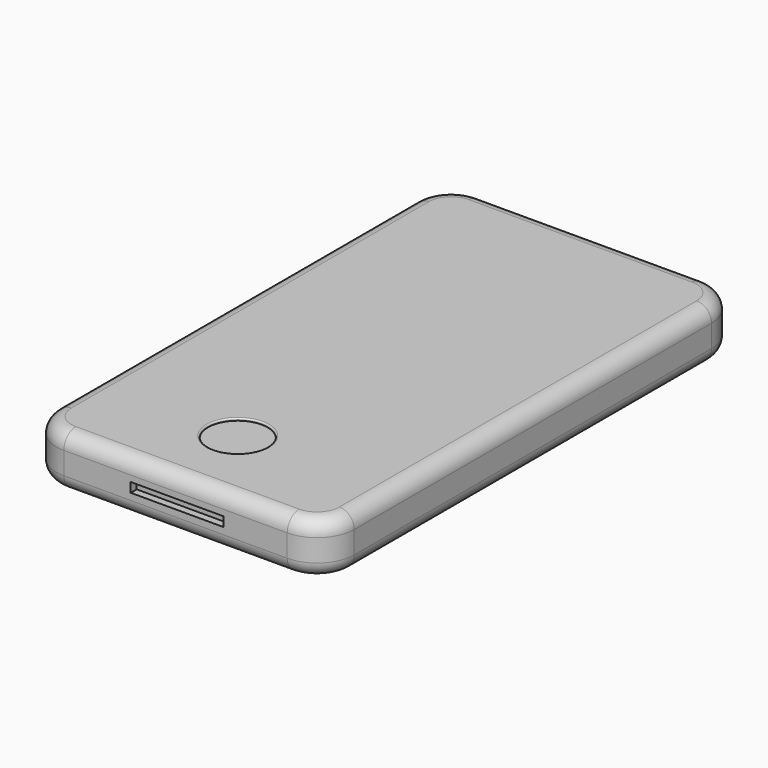
from build123d import *

# Parameters (mm, degrees)
F0_W         = 40
F0_H         = 70
F1_DEPTH     = 7
F2_R         = 5
F3_R         = 2
F4_DEPTH     = 5
F5_T1_DEPTH  = 60
F5_T3_DEPTH  = 30
F5_T6_ANGLE  = 90
F5_T8_ANGLE  = 90
F5_T10_ANGLE = 90
F5_T12_ANGLE = 90
F5_T14_ANGLE = 90
F5_T16_ANGLE = 90
F5_T18_ANGLE = 90
F5_T20_ANGLE = 90
F6_R         = 4
F7_DEPTH     = 0.3
F8_R         = 0.2
F9_W         = 12.4906748533
F9_H         = 1.2735207565
F10_DEPTH    = 1


# Not quite as in the source:
# - a fillet or chamfer that OpenCascade refuses, or shapes differently, is made with other operations: its cross-section is extruded or revolved along the edge and cut away or added


with BuildPart() as f1:
    # F0 (on Top) → F1 (new body)
    with BuildSketch(Plane.XY):
        with Locations((20, 35)):
            Rectangle(F0_W, F0_H)
    extrude(amount=F1_DEPTH)

    # F2
    f2_edges = [f1.edges().sort_by_distance(p)[0] for p in [
        (40, 0, 3.5),
        (0, 0, 3.5),
        (40, 70, 3.5),
        (0, 70, 3.5),
    ]]
    fillet(f2_edges, radius=F2_R)

    # F3 (on face) → F4 (cut)
    with BuildSketch(Plane(origin=(0, 70, 0), x_dir=(-1, 0, 0), z_dir=(0, 1, 0))):
        with Locations((-30.8697689325, 3.5)):
            Circle(F3_R)
    extrude(amount=-F4_DEPTH, mode=Mode.SUBTRACT)

    # F5: fillet of radius 2 on 16 edges, made by hand

    # F5_s2 → F5_t1 (cut)
    with BuildSketch(Plane.XZ.offset(-65)):
        with BuildLine():
            ThreePointArc((0, 5), (0.5857864376, 6.4142135624), (2, 7))
            Line((2, 7), (0, 7))
            Line((0, 7), (0, 5))
        make_face()
        with BuildLine():
            ThreePointArc((38, 7), (39.4142135624, 6.4142135624), (40, 5))
            Line((40, 5), (40, 7))
            Line((40, 7), (38, 7))
        make_face()
        with BuildLine():
            ThreePointArc((0, 2), (0.5857864376, 0.5857864376), (2, 0))
            Line((2, 0), (0, 0))
            Line((0, 0), (0, 2))
        make_face()
        with BuildLine():
            ThreePointArc((38, 0), (39.4142135624, 0.5857864376), (40, 2))
            Line((40, 2), (40, 0))
            Line((40, 0), (38, 0))
        make_face()
    extrude(amount=F5_T1_DEPTH, mode=Mode.SUBTRACT)

    # F5_s4 → F5_t3 (cut)
    with BuildSketch(Plane.YZ.offset(5)):
        with BuildLine():
            ThreePointArc((68, 7), (69.4142135624, 6.4142135624), (70, 5))
            Line((70, 5), (70, 7))
            Line((70, 7), (68, 7))
        make_face()
        with BuildLine():
            ThreePointArc((2, 7), (0.5857864376, 6.4142135624), (0, 5))
            Line((0, 5), (0, 7))
            Line((0, 7), (2, 7))
        make_face()
        with BuildLine():
            ThreePointArc((68, 0), (69.4142135624, 0.5857864376), (70, 2))
            Line((70, 2), (70, 0))
            Line((70, 0), (68, 0))
        make_face()
        with BuildLine():
            ThreePointArc((2, 0), (0.5857864376, 0.5857864376), (0, 2))
            Line((0, 2), (0, 0))
            Line((0, 0), (2, 0))
        make_face()
    extrude(amount=F5_T3_DEPTH, mode=Mode.SUBTRACT)

    # F5_s5 → F5_t6 (revolve, cut)
    with BuildSketch(Plane.XZ.offset(-65)):
        with BuildLine():
            ThreePointArc((0, 5), (0.5857864376, 6.4142135624), (2, 7))
            Line((2, 7), (0, 7))
            Line((0, 7), (0, 5))
        make_face()
    revolve(axis=Axis((5, 65, 7), (0, 0, -1)), revolution_arc=F5_T6_ANGLE, mode=Mode.SUBTRACT)

    # F5_s7 → F5_t8 (revolve, cut)
    with BuildSketch(Plane.XZ.offset(-5)):
        with BuildLine():
            ThreePointArc((0, 5), (0.5857864376, 6.4142135624), (2, 7))
            Line((2, 7), (0, 7))
            Line((0, 7), (0, 5))
        make_face()
    revolve(axis=Axis((5, 5, 7), (0, 0, 1)), revolution_arc=F5_T8_ANGLE, mode=Mode.SUBTRACT)

    # F5_s9 → F5_t10 (revolve, cut)
    with BuildSketch(Plane.XZ.offset(-65)):
        with BuildLine():
            ThreePointArc((38, 7), (39.4142135624, 6.4142135624), (40, 5))
            Line((40, 5), (40, 7))
            Line((40, 7), (38, 7))
        make_face()
    revolve(axis=Axis((35, 65, 7), (0, 0, 1)), revolution_arc=F5_T10_ANGLE, mode=Mode.SUBTRACT)

    # F5_s11 → F5_t12 (revolve, cut)
    with BuildSketch(Plane.YZ.offset(35)):
        with BuildLine():
            ThreePointArc((2, 7), (0.5857864376, 6.4142135624), (0, 5))
            Line((0, 5), (0, 7))
            Line((0, 7), (2, 7))
        make_face()
    revolve(axis=Axis((35, 5, 7), (0, 0, 1)), revolution_arc=F5_T12_ANGLE, mode=Mode.SUBTRACT)

    # F5_s13 → F5_t14 (revolve, cut)
    with BuildSketch(Plane.XZ.offset(-65)):
        with BuildLine():
            ThreePointArc((2, 0), (0.5857864376, 0.5857864376), (0, 2))
            Line((0, 2), (0, 0))
            Line((0, 0), (2, 0))
        make_face()
    revolve(axis=Axis((5, 65, 0), (0, 0, -1)), revolution_arc=F5_T14_ANGLE, mode=Mode.SUBTRACT)

    # F5_s15 → F5_t16 (revolve, cut)
    with BuildSketch(Plane.XZ.offset(-5)):
        with BuildLine():
            ThreePointArc((2, 0), (0.5857864376, 0.5857864376), (0, 2))
            Line((0, 2), (0, 0))
            Line((0, 0), (2, 0))
        make_face()
    revolve(axis=Axis((5, 5, 0), (0, 0, 1)), revolution_arc=F5_T16_ANGLE, mode=Mode.SUBTRACT)

    # F5_s17 → F5_t18 (revolve, cut)
    with BuildSketch(Plane.XZ.offset(-65)):
        with BuildLine():
            ThreePointArc((38, 0), (39.4142135624, 0.5857864376), (40, 2))
            Line((40, 2), (40, 0))
            Line((40, 0), (38, 0))
        make_face()
    revolve(axis=Axis((35, 65, 0), (0, 0, 1)), revolution_arc=F5_T18_ANGLE, mode=Mode.SUBTRACT)

    # F5_s19 → F5_t20 (revolve, cut)
    with BuildSketch(Plane.YZ.offset(35)):
        with BuildLine():
            ThreePointArc((2, 0), (0.5857864376, 0.5857864376), (0, 2))
            Line((0, 2), (0, 0))
            Line((0, 0), (2, 0))
        make_face()
    revolve(axis=Axis((35, 5, 0), (0, 0, 1)), revolution_arc=F5_T20_ANGLE, mode=Mode.SUBTRACT)

    # F6 (on face) → F7 (cut)
    with BuildSketch(Plane.XY.offset(7)):
        with Locations((19.5677466691, 10.9801534563)):
            Circle(F6_R)
    extrude(amount=-F7_DEPTH, mode=Mode.SUBTRACT)

    # F8
    f8_edges = [f1.edges().sort_by_distance(p)[0] for p in [
        (15.567747, 10.980153, 7),
        (2.87868, 67.12132, 7),
        (2, 35, 7),
        (20, 68, 7),
        (2.87868, 2.87868, 7),
        (37.12132, 67.12132, 7),
        (20, 2, 7),
        (38, 35, 7),
        (37.12132, 2.87868, 7),
    ]]
    fillet(f8_edges, radius=F8_R)

    # F9 (on face) → F10 (cut)
    with BuildSketch(Plane.XZ):
        with Locations((20.2241037041, 3.5419908818)):
            Rectangle(F9_W, F9_H)
    extrude(amount=-F10_DEPTH, mode=Mode.SUBTRACT)


solid = f1.part
